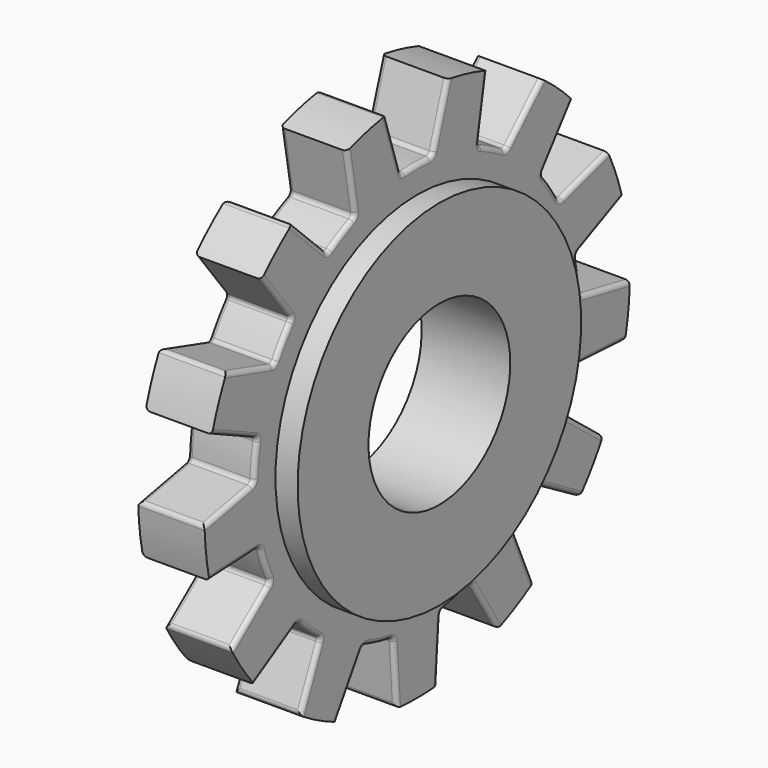
from build123d import *

# Parameters (mm, degrees)
F3_DEPTH        = 25.4
F3_COPIES_COUNT = 13
F4_R            = 1.27


# Not quite as in the source:
# - a feature of the source that left no trace in its solid (it failed there, or was rolled back) is left out
# - a pattern or mirror of a feature is missing from the dataset's text; its kind, count and spacing are read off the source's solid


with BuildPart() as f1:
    # F0 (on Front) → F1 (revolve)
    with BuildSketch(Plane.XZ):
        Polygon((-22.2074580775, 25.4), (-41.2574580775, 25.4), (-41.2574580775, -25.4), (-15.8574580775, -25.4), (-15.8574580775, 0), (-22.2074580775, 0), align=None)
    revolve(axis=Axis((-20.5299006775, 0, -50.8), (1, 0, 0)))

    # F2 (on face) → F3 (cut)
    with BuildSketch(Plane.YZ.offset(-22.2074580775)):
        with BuildLine():
            ThreePointArc((11.0854199288, 24.5893458322), (0, 25.4), (-11.0854199288, 24.5893458322))
            Line((-11.0854199288, 24.5893458322), (-5.5259202022, 7.3712119068))
            ThreePointArc((-5.5259202022, 7.3712119068), (0, 7.6330872776), (5.5259202022, 7.3712119068))
            Line((5.5259202022, 7.3712119068), (11.0854199288, 24.5893458322))
        make_face()
    f3 = extrude(amount=-F3_DEPTH, mode=Mode.SUBTRACT)

    # F3_copies: F3 ×13 about axis
    f3_copies_axis = Axis((0, 0, -50.8), (1, 0, 0))
    for i in range(1, F3_COPIES_COUNT):
        add(f3.rotate(f3_copies_axis, i * 360 / F3_COPIES_COUNT), mode=Mode.SUBTRACT)

    # F4
    f4_edges = [f1.edges().sort_by_distance(p)[0] for p in [
        (-22.207458, -8.30567, 15.980279),
        (-31.732458, -5.52592, 7.371212),
        (-41.257458, -8.30567, 15.980279),
        (-31.732458, -11.08542, 24.589346),
        (-22.207458, 0, 7.633087),
        (-31.732458, 5.52592, 7.371212),
        (-41.257458, 0, 7.633087),
        (-41.257458, 8.30567, 15.980279),
        (-41.257458, 23.680037, 12.190838),
        (-41.257458, 27.15521, 0.939929),
        (-41.257458, 38.388649, 4.471163),
        (-41.257458, 50.240934, -6.029045),
        (-41.257458, 48.089488, -17.606223),
        (-41.257458, 59.67725, -19.69991),
        (-41.257458, 65.292238, -34.505414),
        (-41.257458, 58.007044, -43.75667),
        (-41.257458, 67.294513, -50.995639),
        (-41.257458, 65.385877, -66.714677),
        (-41.257458, 54.635886, -71.520658),
        (-41.257458, 59.495414, -82.24655),
        (-41.257458, 50.500399, -95.278078),
        (-41.257458, 38.748304, -94.537794),
        (-41.257458, 38.066633, -106.293435),
        (-41.257458, 24.045889, -113.652088),
        (-41.257458, 13.983953, -107.535128),
        (-41.257458, 7.917244, -117.627442),
        (-41.257458, -7.917244, -117.627442),
        (-41.257458, -13.983953, -107.535128),
        (-41.257458, -24.045889, -113.652088),
        (-41.257458, -38.066633, -106.293435),
        (-41.257458, -38.748304, -94.537794),
        (-41.257458, -50.500399, -95.278078),
        (-41.257458, -59.495414, -82.24655),
        (-41.257458, -54.635886, -71.520658),
        (-41.257458, -65.385877, -66.714677),
        (-41.257458, -67.294513, -50.995639),
        (-41.257458, -58.007044, -43.75667),
        (-41.257458, -65.292238, -34.505414),
        (-41.257458, -59.67725, -19.69991),
        (-41.257458, -48.089488, -17.606223),
        (-41.257458, -50.240934, -6.029045),
        (-41.257458, -38.388649, 4.471163),
        (-41.257458, -27.15521, 0.939929),
        (-41.257458, -23.680037, 12.190838),
        (-22.207458, -23.680037, 12.190838),
        (-31.732458, -22.140551, 3.276073),
        (-22.207458, -27.15521, 0.939929),
        (-22.207458, -38.388649, 4.471163),
        (-22.207458, -50.240934, -6.029045),
        (-22.207458, -48.089488, -17.606223),
        (-22.207458, -59.67725, -19.69991),
        (-22.207458, -65.292238, -34.505414),
        (-22.207458, -58.007044, -43.75667),
        (-22.207458, -67.294513, -50.995639),
        (-22.207458, -65.385877, -66.714677),
        (-22.207458, -54.635886, -71.520658),
        (-22.207458, -59.495414, -82.24655),
        (-22.207458, -50.500399, -95.278078),
        (-22.207458, -38.748304, -94.537794),
        (-22.207458, -38.066633, -106.293435),
        (-22.207458, -24.045889, -113.652088),
        (-22.207458, -13.983953, -107.535128),
        (-22.207458, -7.917244, -117.627442),
        (-22.207458, 7.917244, -117.627442),
        (-22.207458, 13.983953, -107.535128),
        (-22.207458, 24.045889, -113.652088),
        (-22.207458, 38.066633, -106.293435),
        (-22.207458, 38.748304, -94.537794),
        (-22.207458, 50.500399, -95.278078),
        (-22.207458, 59.495414, -82.24655),
        (-22.207458, 54.635886, -71.520658),
        (-22.207458, 65.385877, -66.714677),
        (-22.207458, 67.294513, -50.995639),
        (-22.207458, 58.007044, -43.75667),
        (-22.207458, 65.292238, -34.505414),
        (-22.207458, 59.67725, -19.69991),
        (-22.207458, 48.089488, -17.606223),
        (-22.207458, 50.240934, -6.029045),
        (-22.207458, 38.388649, 4.471163),
        (-22.207458, 27.15521, 0.939929),
        (-22.207458, 23.680037, 12.190838),
        (-22.207458, 8.30567, 15.980279),
        (-31.732458, 25.219524, 21.105602),
        (-31.732458, 22.140551, 3.276073),
        (-31.732458, 31.926469, -1.859973),
        (-31.732458, 55.746979, 1.149151),
        (-31.732458, 44.734888, -13.207242),
        (-31.732458, 51.013049, -22.302728),
        (-31.732458, 73.503473, -30.708224),
        (-31.732458, 57.081002, -38.302605),
        (-31.732458, 58.413154, -49.273865),
        (-31.732458, 74.421207, -67.168383),
        (-31.732458, 56.350546, -66.260971),
        (-31.732458, 52.43151, -76.594621),
        (-31.732458, 58.289939, -99.878743),
        (-31.732458, 42.710859, -90.677414),
        (-31.732458, 34.438438, -98.00614),
        (-31.732458, 28.805149, -121.345754),
        (-31.732458, 19.286629, -105.958423),
        (-31.732458, 8.555935, -108.603301),
        (-31.732458, -7.278554, -126.651583),
        (-31.732458, -8.555935, -108.603301),
        (-31.732458, -19.286629, -105.958423),
        (-31.732458, -41.694827, -114.580729),
        (-31.732458, -34.438438, -98.00614),
        (-31.732458, -42.710859, -90.677414),
        (-31.732458, -66.559319, -87.898478),
        (-31.732458, -52.43151, -76.594621),
        (-31.732458, -56.350546, -66.260971),
        (-31.732458, -76.175872, -52.717413),
        (-31.732458, -58.413154, -49.273865),
        (-31.732458, -57.081002, -38.302605),
        (-31.732458, -68.341452, -17.097092),
        (-31.732458, -51.013049, -22.302728),
        (-31.732458, -44.734888, -13.207242),
        (-31.732458, -44.850828, 10.802299),
        (-31.732458, -31.926469, -1.859973),
    ]]
    fillet(f4_edges, radius=F4_R)


solid = f1.part
